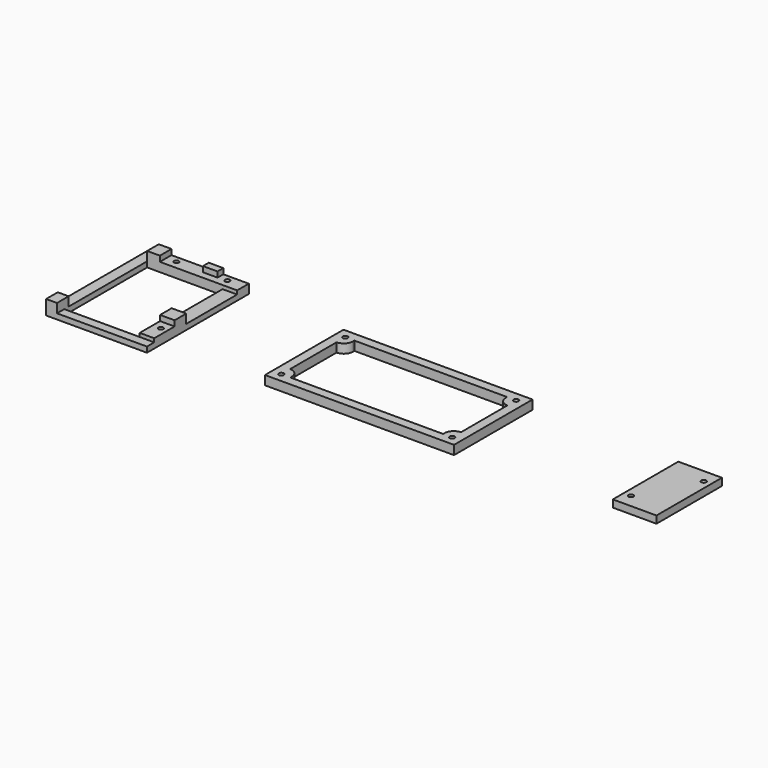
from build123d import *

# Parameters (mm, degrees)
F0_W      = 104
F0_H      = 54
F1_DEPTH  = 5
F2_R      = 1.35
F3_DEPTH  = 3.5
F4_R      = 4.99999
F5_W      = 24
F5_H      = 45
F5_R      = 1.35
F6_DEPTH  = 4
F7_W      = 55.5
F7_H      = 70
F7_W_2    = 41.5
F7_H_2    = 57
F8_DEPTH  = 5
F9_W      = 7
F9_H      = 8
F9_W_2    = 8
F9_H_2    = 4
F9_W_3    = 6
F10_DEPTH = 3
F12_W     = 6
F12_H     = 62
F12_W_2   = 49.5
F12_H_2   = 5
F12_W_3   = 8
F12_H_3   = 35
F13_DEPTH = 2
F14_R     = 1.3
F15_DEPTH = 4


# Not quite as in the source:
# - a fillet or chamfer is up to 0.001 mm smaller than in the source, because OpenCascade refuses the exact size


with BuildPart() as f1:
    # F0 (on Top) → F1 (new body)
    with BuildSketch(Plane.XY):
        Rectangle(F0_W, F0_H)
        Polygon((-42, 16), (-42, 22), (42, 22), (42, 16), (47, 16), (47, -16), (42, -16), (42, -22), (-42, -22), (-42, -16), (-47, -16), (-47, 16), align=None, mode=Mode.SUBTRACT)
    extrude(amount=F1_DEPTH)

    # F2 (on face) → F3 (cut)
    with BuildSketch(Plane.XY.offset(5)):
        with Locations((-47, 22)):
            Circle(F2_R)
        with Locations((47, 22)):
            Circle(F2_R)
        with Locations((-47, -22)):
            Circle(F2_R)
        with Locations((47, -22)):
            Circle(F2_R)
    extrude(amount=-F3_DEPTH, mode=Mode.SUBTRACT)

    # F4 (radius 5 in the source; OpenCascade refuses exactly that, so slightly less here)
    f4_edges = [f1.edges().sort_by_distance(p)[0] for p in [
        (-42, 16, 2.5),
        (-42, -16, 2.5),
        (42, 16, 2.5),
        (42, -16, 2.5),
    ]]
    fillet(f4_edges, radius=F4_R)


with BuildPart() as f6:
    # F5 (on Top) → F6 (new body)
    with BuildSketch(Plane.XY):
        with Locations((147.7760076523, 0)):
            Rectangle(F5_W, F5_H)
        with Locations((139.7760076523, -15)):
            Circle(F5_R, mode=Mode.SUBTRACT)
        with Locations((155.7760076523, 15)):
            Circle(F5_R, mode=Mode.SUBTRACT)
    extrude(amount=F6_DEPTH)


with BuildPart() as f8:
    # F7 (on Top) → F8 (new body)
    with BuildSketch(Plane.XY):
        with Locations((-138.2528990507, 0)):
            Rectangle(F7_W, F7_H)
        with Locations((-139.2528990507, -1.5)):
            Rectangle(F7_W_2, F7_H_2, mode=Mode.SUBTRACT)
    extrude(amount=F8_DEPTH)

    # F9 (on face) → F10 (join)
    with BuildSketch(Plane.XY.offset(5)):
        with Locations((-156.5028990507, 31)):
            Rectangle(F9_W, F9_H)
        with Locations((-128.5028990507, 33)):
            Rectangle(F9_W_2, F9_H_2)
        with Locations((-114.5028990507, -12)):
            Rectangle(F9_W_2, F9_H)
        with Locations((-163.0028990507, -31)):
            Rectangle(F9_W_3, F9_H)
    extrude(amount=F10_DEPTH)

    # F12 (on offset) → F13 (cut)
    with BuildSketch(Plane.XY.offset(5)):
        with Locations((-163.0028990507, 4)):
            Rectangle(F12_W, F12_H)
        with Locations((-135.2528990507, -32.5)):
            Rectangle(F12_W_2, F12_H_2)
        with Locations((-114.5028990507, 9.5)):
            Rectangle(F12_W_3, F12_H_3)
    extrude(amount=-F13_DEPTH, mode=Mode.SUBTRACT)

    # F14 (on face) → F15 (cut)
    with BuildSketch(Plane.XY.offset(5)):
        with Locations((-147.5028990507, 31.5)):
            Circle(F14_R)
        with Locations((-119.5028990507, 31.5)):
            Circle(F14_R)
        with Locations((-114.0028990507, -21)):
            Circle(F14_R)
    extrude(amount=-F15_DEPTH, mode=Mode.SUBTRACT)


solid = Compound([f1.part, f6.part, f8.part])
